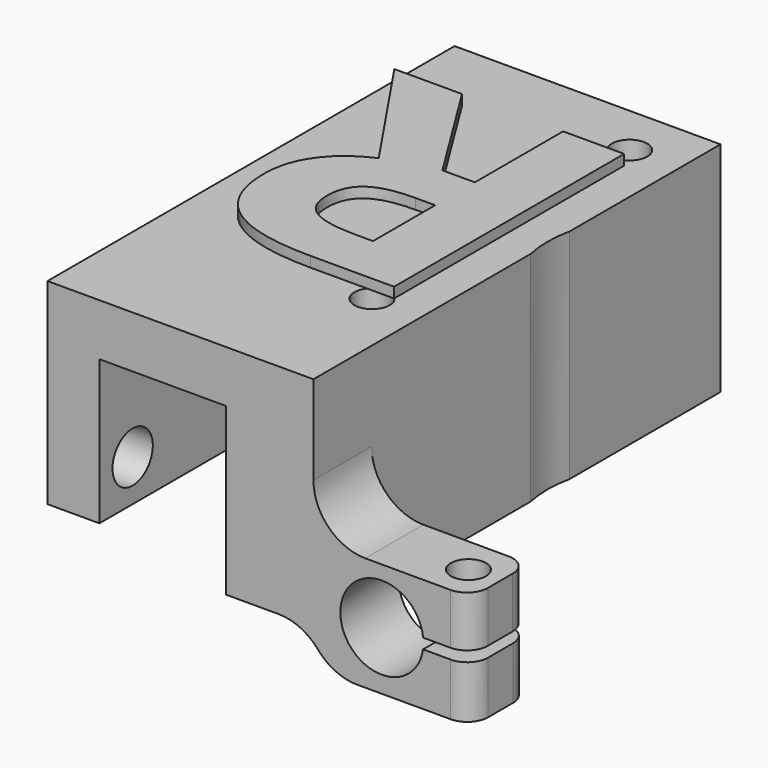
from build123d import *

# Parameters (mm, degrees)
F1_DEPTH      = 7
F2_DEPTH      = 42
F3_R          = 1.7
F3_R_2        = 11
F4_DEPTH      = 21.001
F5_R          = 4
F6_DEPTH      = 10
F7_DEPTH      = 21.001
F8_R          = 1.4
F9_DEPTH      = 11.0207610561
F8_R_2        = 1.7
F10_DEPTH     = 4.9110969969
F11_R         = 5
F12_R         = 5
F13_R         = 5
F14_R         = 2
F15_R         = 2.2
F15_R_2       = 2.4255023423
F16_DEPTH     = 6
F17_TEXT_SIZE = 38.7940819345
F18_DEPTH     = 1


# Not quite as in the source:
# - a feature names something its author has since deleted; it is built from what else it names
# - Text() gives the source's letters only with a copy of the font that has no kerning and outlines rounded to 1/6400 em; it was checked with that copy


with BuildPart() as f1:
    # F0 (on Front) → F1 (new body)
    with BuildSketch(Plane.XZ):
        Polygon((-18.6721007523, 29.8099789735), (-18.6721007523, 10.8925135386), (-13.6721007523, 10.8925135386), (-13.6721007523, 24.8099789735), (-1.4721007523, 24.8099789735), (-1.4721007523, 8.8099789735), (6.9380548998, 8.8099789735), (6.9380548998, 16.2656020473), (6.9380548998, 29.8099789735), align=None)
        Polygon((22.1263195603, 16.2417280634), (6.9380548998, 16.2656020473), (6.9380548998, 8.8099789735), (8.3533044869, 5.2860832236), (22.1553367778, 5.2860832236), (22.1553367778, 10.343908232), (15.4860510706, 10.343908232), (15.4860510706, 11.3388913612), (22.1263195603, 11.3388913612), align=None)
    extrude(amount=F1_DEPTH)

    # F0 (on Front) → F2 (join)
    with BuildSketch(Plane.XZ):
        Polygon((-18.6721007523, 29.8099789735), (-18.6721007523, 10.8925135386), (-13.6721007523, 10.8925135386), (-13.6721007523, 24.8099789735), (-1.4721007523, 24.8099789735), (-1.4721007523, 8.8099789735), (6.9380548998, 8.8099789735), (6.9380548998, 16.2656020473), (6.9380548998, 29.8099789735), align=None)
    extrude(amount=-F2_DEPTH)

    # F3 (on face) → F4 (cut, through all)
    with BuildSketch(Plane(origin=(0, 0, 8.8099789735), x_dir=(1, 0, 0), z_dir=(0, 0, -1))):
        with Locations((2.1850741468, -6)):
            Circle(F3_R)
        with Locations((2.1850741468, -37)):
            Circle(F3_R)
        with Locations((17.6850741468, -21.5)):
            Circle(F3_R_2)
    extrude(amount=-F4_DEPTH, mode=Mode.SUBTRACT)

    # F5 (on face) → F6 (cut)
    with BuildSketch(Plane.XZ.offset(7)):
        with Locations((13.5278992477, 10.8989789735)):
            Circle(F5_R)
    extrude(amount=-F6_DEPTH, mode=Mode.SUBTRACT)

    # F3 (on face) → F7 (cut, through all)
    with BuildSketch(Plane(origin=(0, 0, 8.8099789735), x_dir=(1, 0, 0), z_dir=(0, 0, -1))):
        with Locations((2.1850741468, -6)):
            Circle(F3_R)
        with Locations((2.1850741468, -37)):
            Circle(F3_R)
        with Locations((17.6850741468, -21.5)):
            Circle(F3_R_2)
    extrude(amount=-F7_DEPTH, mode=Mode.SUBTRACT)

    # F8 (on face) → F9 (cut, through all)
    with BuildSketch(Plane(origin=(0.0255844979, 0, 16.2764675551), x_dir=(0.9999987646, 0, -0.0015718685), z_dir=(0.0015718685, 0, 0.9999987646))):
        with Locations((19.1007623654, -3.5767070949)):
            Circle(F8_R)
    extrude(amount=-F9_DEPTH, mode=Mode.SUBTRACT)

    # F8 (on face) → F10 (cut, through all)
    with BuildSketch(Plane(origin=(0.0255844979, 0, 16.2764675551), x_dir=(0.9999987646, 0, -0.0015718685), z_dir=(0.0015718685, 0, 0.9999987646))):
        with Locations((19.1007623654, -3.5767070949)):
            Circle(F8_R_2)
        with Locations((19.1007623654, -3.5767070949)):
            Circle(F8_R, mode=Mode.SUBTRACT)
    extrude(amount=-F10_DEPTH, mode=Mode.SUBTRACT)

    # F11
    f11_edges = [f1.edges().sort_by_distance(p)[0] for p in [
        (6.938055, -3.5, 16.265602),
    ]]
    fillet(f11_edges, radius=F11_R)

    # F12
    f12_edges = [f1.edges().sort_by_distance(p)[0] for p in [
        (6.938055, -3.5, 8.809979),
    ]]
    fillet(f12_edges, radius=F12_R)

    # F13
    f13_edges = [f1.edges().sort_by_distance(p)[0] for p in [
        (8.353304, -3.5, 5.286083),
    ]]
    fillet(f13_edges, radius=F13_R)

    # F14
    f14_edges = [f1.edges().sort_by_distance(p)[0] for p in [
        (22.12632, -7, 13.79031),
        (22.155337, -7, 7.814996),
        (22.12632, 0, 13.79031),
        (22.155337, 0, 7.814996),
    ]]
    fillet(f14_edges, radius=F14_R)

    # F15 (on face) → F16 (cut)
    with BuildSketch(Plane(origin=(-18.6721007523, 0, 0), x_dir=(0, -1, 0), z_dir=(-1, 0, 0))):
        with Locations((-38, 14.8925135386)):
            Circle(F15_R)
        with Locations((3, 14.8925135386)):
            Circle(F15_R_2)
    extrude(amount=-F16_DEPTH, mode=Mode.SUBTRACT)

    # F17 (on face) → F18 (join)
    with BuildSketch(Plane.XY.offset(29.8099789735)):
        with Locations(Location((6.9380548998, 34.7543930674), (0, 0, 180))):
            Text('R', F17_TEXT_SIZE, font='Open Sans', font_style=FontStyle.BOLD, text_align=(TextAlign.LEFT, TextAlign.BOTTOM))
    extrude(amount=F18_DEPTH)


solid = f1.part
